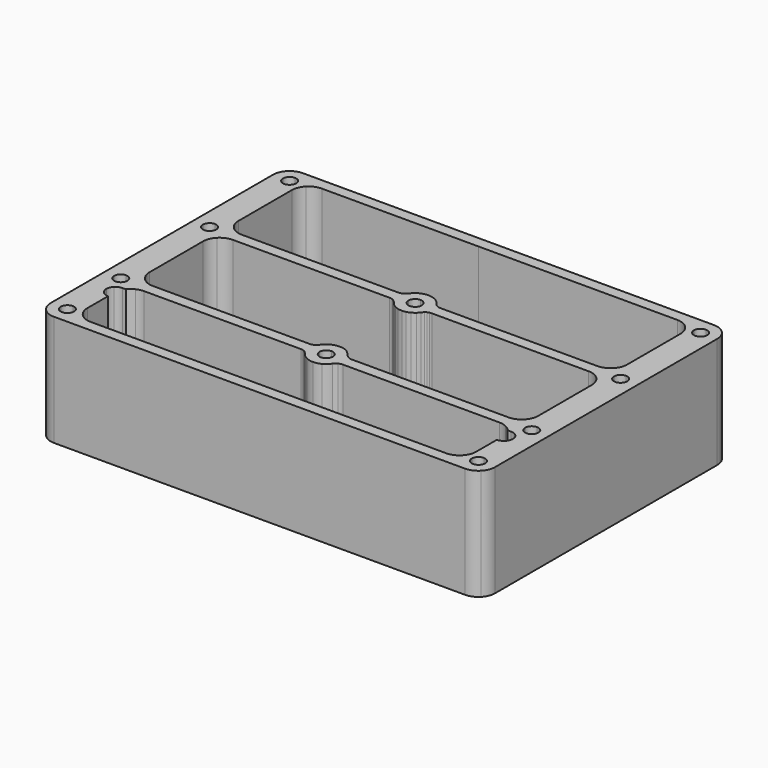
from build123d import *

# Parameters (mm, degrees)
F1_DEPTH = 20


# Not quite as in the source:
# - ends of sketch curves that miss each other by under 0.0002 mm in the source are joined


with BuildPart() as f1:
    # F0 (on Top) → F1 (new body)
    with BuildSketch(Plane.XY):
        with BuildLine():
            Line((-39.999825, 25.00006), (-39.999825, -24.99994))
            Line((-39.999825, -24.99994), (-40.000174, -25.00006))
            ThreePointArc((-40.000174, -25.00006), (-39.771812164, -26.1481105372), (-39.1214940862, -27.1213810862))
            ThreePointArc((-39.1214940862, -27.1213810862), (-38.1480375077, -27.7716732647), (-36.999825, -27.9999399831))
            Line((-36.999825, -27.9999399831), (36.999826, -28.00006))
            ThreePointArc((36.999826, -28.00006), (38.1478759832, -27.7716986429), (39.121146172, -27.121381172))
            ThreePointArc((39.121146172, -27.121381172), (39.7716506494, -26.1480852785), (40.000174978, -24.99994))
            Line((40.000174978, -24.99994), (39.999826, 24.99994))
            ThreePointArc((39.999826, 24.99994), (39.7714639135, 26.1479899431), (39.1211458791, 27.1212598791))
            ThreePointArc((39.1211458791, 27.1212598791), (38.1480624616, 27.7716033194), (37.000175, 28.0000599827))
            Line((37.000175, 28.0000599827), (-37.000174, 27.99994))
            ThreePointArc((-37.000174, 27.99994), (-38.1482239431, 27.7715779135), (-39.1214938791, 27.1212598791))
            ThreePointArc((-39.1214938791, 27.1212598791), (-39.7716257147, 26.1480153964), (-39.999825, 25.00006))
        make_face()
        with BuildLine():
            Line((-38.200174, -24.99956), (-38.199825, -24.99994))
            ThreePointArc((-38.1998249445, -24.99994), (-37.8486064453, -24.1512940355), (-37.000174, -23.7995600552))
            ThreePointArc((-37.000174, -23.79956), (-36.1516455697, -24.1510315697), (-35.800174, -24.99956))
            ThreePointArc((-35.800174, -24.99956), (-36.1516455697, -25.8480884303), (-37.000174, -26.19956))
            ThreePointArc((-37.000174, -26.19956), (-37.8487024303, -25.8480884303), (-38.200174, -24.99956))
        make_face(mode=Mode.SUBTRACT)
        with BuildLine():
            Line((-38.200174, -12.99956), (-38.199825, -12.99994))
            ThreePointArc((-38.1998249445, -12.99994), (-37.8486064453, -12.1512940355), (-37.000174, -11.7995600552))
            ThreePointArc((-37.000174, -11.79956), (-36.1516455697, -12.1510315697), (-35.800174, -12.99956))
            ThreePointArc((-35.800174, -12.99956), (-36.1516455697, -13.8480884303), (-37.000174, -14.19956))
            ThreePointArc((-37.000174, -14.19956), (-37.8487024303, -13.8480884303), (-38.200174, -12.99956))
        make_face(mode=Mode.SUBTRACT)
        with BuildLine():
            Line((-1.200174, -12.99956), (-1.199825, -12.99994))
            ThreePointArc((-1.1998249445, -12.99994), (-0.8486064453, -12.1512940355), (-0.000174, -11.7995600552))
            ThreePointArc((-0.000174, -11.79956), (0.8483544303, -12.1510315697), (1.199826, -12.99956))
            ThreePointArc((1.199826, -12.99956), (0.8483544303, -13.8480884303), (-0.000174, -14.19956))
            ThreePointArc((-0.000174, -14.19956), (-0.8487024303, -13.8480884303), (-1.200174, -12.99956))
        make_face(mode=Mode.SUBTRACT)
        with BuildLine():
            Line((36.603538, -16.75006), (36.603175, -16.74994))
            ThreePointArc((36.603175, -16.74994), (36.4829333909, -17.3619187603), (36.1383180086, -17.8817420086))
            ThreePointArc((36.1383180086, -17.8817420086), (35.6165430962, -18.2356135959), (34.9998259968, -18.3665107942))
            Line((34.9998259968, -18.3665107942), (35.000175, -22.99994))
            ThreePointArc((35.000175, -22.99994), (34.7716506494, -24.1480852785), (34.121146138, -25.1213811381))
            ThreePointArc((34.121146138, -25.1213811381), (33.1478759832, -25.7716986429), (31.999826, -26.00006))
            Line((31.999826, -26.00006), (-31.999825, -25.99994))
            ThreePointArc((-31.999825, -25.99994), (-33.1480375077, -25.7716732647), (-34.1214941324, -25.1213811324))
            ThreePointArc((-34.1214941324, -25.1213811324), (-34.771812164, -24.1481105372), (-35.000174, -23.00006))
            Line((-35.000174, -23.00006), (-34.999825, -18.34994))
            ThreePointArc((-34.999825, -18.34994), (-35.6042335809, -18.2304702332), (-36.1159159305, -17.887302931))
            ThreePointArc((-36.1159159305, -17.887302931), (-36.4642279095, -17.3651332541), (-36.5893969659, -16.7500599998))
            ThreePointArc((-36.5893969659, -16.7500599998), (-36.4636878106, -16.133963155), (-36.1146695958, -15.6109294015))
            ThreePointArc((-36.1146695958, -15.6109294015), (-35.6037340191, -15.2685004223), (-35.0001739964, -15.1500592171))
            Line((-35.0001739964, -15.1500592171), (-34.373825, -15.14994))
            ThreePointArc((-34.373825, -15.14994), (-33.8806261156, -14.6647208591), (-33.2945678918, -14.297000223))
            ThreePointArc((-33.2945678918, -14.297000223), (-32.6642661787, -14.074224434), (-32.0001739998, -13.9974720891))
            Line((-32.0001739998, -13.9974720891), (-3.792825, -13.99294))
            ThreePointArc((-3.792825, -13.99294), (-3.587024283, -14.0085288519), (-3.3845238859, -14.0484105604))
            ThreePointArc((-3.3845238859, -14.0484105604), (-3.1995526999, -14.1089426612), (-3.0236719787, -14.1922759616))
            ThreePointArc((-3.0236719787, -14.1922759616), (-2.8987221408, -14.2721320584), (-2.7848178748, -14.3670808678))
            ThreePointArc((-2.7848178748, -14.3670808678), (-2.6072336828, -14.548031177), (-2.4434346201, -14.7415487017))
            ThreePointArc((-2.4434346201, -14.7415487017), (-1.9532323269, -15.2735515805), (-1.3530931568, -15.6774803045))
            ThreePointArc((-1.3530931568, -15.6774803045), (-0.6961967844, -15.9206969026), (-0.0001739951, -15.999560602))
            ThreePointArc((-0.0001739951, -15.999560602), (0.7201727666, -15.9154593612), (1.3979399526, -15.6573819105))
            ThreePointArc((1.3979399526, -15.6573819105), (1.982334578, -15.2460332249), (2.4460271812, -14.7022374632))
            ThreePointArc((2.4460271812, -14.7022374632), (2.7407409968, -14.4052400968), (3.089711319, -14.1744086099))
            ThreePointArc((3.089711319, -14.1744086099), (3.4350131482, -14.0422107565), (3.8014919924, -13.9931905443))
            Line((3.8014919924, -13.9931905443), (32.000175, -13.99994))
            ThreePointArc((32.000175, -13.99994), (32.6691048373, -14.0761652682), (33.3038019175, -14.3007471693))
            ThreePointArc((33.3038019175, -14.3007471693), (33.8771769518, -14.664706996), (34.3550597723, -15.1472561797))
            Line((34.3550597723, -15.1472561797), (35.003175, -15.14994))
            ThreePointArc((35.003175, -15.14994), (35.6171587026, -15.2707727015), (36.1376999935, -15.6180670065))
            ThreePointArc((36.1376999935, -15.6180670065), (36.4838802077, -16.1374542064), (36.603538, -16.75006))
        make_face(mode=Mode.SUBTRACT)
        with BuildLine():
            Line((35.799826, -24.99956), (35.800175, -24.99994))
            ThreePointArc((35.8001750555, -24.99994), (36.1513935547, -24.1512940355), (36.999826, -23.7995600552))
            ThreePointArc((36.999826, -23.79956), (37.8483544303, -24.1510315697), (38.199826, -24.99956))
            ThreePointArc((38.199826, -24.99956), (37.8483544303, -25.8480884303), (36.999826, -26.19956))
            ThreePointArc((36.999826, -26.19956), (36.1512975697, -25.8480884303), (35.799826, -24.99956))
        make_face(mode=Mode.SUBTRACT)
        with BuildLine():
            Line((34.999826, 2.99994), (35.000175, 3.00006))
            Line((35.000175, 3.00006), (35.000175, -8.99994))
            ThreePointArc((35.000175, -8.99994), (34.7716506494, -10.1480852785), (34.121146138, -11.1213811381))
            ThreePointArc((34.121146138, -11.1213811381), (33.1478759832, -11.7716986429), (31.999826, -12.00006))
            Line((31.999826, -12.00006), (3.810175, -11.99994))
            ThreePointArc((3.810175, -11.99994), (3.4730610862, -11.9616796532), (3.1530679652, -11.8489230717))
            ThreePointArc((3.1530679652, -11.8489230717), (2.833800561, -11.6515843202), (2.5610064723, -11.3937905925))
            ThreePointArc((2.5610064723, -11.3937905925), (2.3088636351, -11.0955933493), (2.037311876, -10.8149561283))
            ThreePointArc((2.037311876, -10.8149561283), (1.8071893103, -10.6107695316), (1.5605320798, -10.4268978829))
            ThreePointArc((1.5605320798, -10.4268978829), (1.4100194875, -10.3334911747), (1.2521070594, -10.2532258697))
            ThreePointArc((1.2521070594, -10.2532258697), (1.064969326, -10.1762092608), (0.8726172571, -10.1133381012))
            ThreePointArc((0.8726172571, -10.1133381012), (0.6668393246, -10.0626764147), (0.4578610603, -10.0274735375))
            ThreePointArc((0.4578610603, -10.0274735375), (0.2293235598, -10.0056398158), (-0.000173999, -9.9995601312))
            ThreePointArc((-0.000173999, -9.9995601312), (-0.7183583445, -10.0837537005), (-1.3940161851, -10.3413656513))
            ThreePointArc((-1.3940161851, -10.3413656513), (-2.0176152889, -10.7733522055), (-2.5231648411, -11.3389561115))
            ThreePointArc((-2.5231648411, -11.3389561115), (-2.7518538477, -11.6084835939), (-3.0417751614, -11.81069469))
            ThreePointArc((-3.0417751614, -11.81069469), (-3.4064030036, -11.949362238), (-3.7931999932, -12.0000604896))
            Line((-3.7931999932, -12.0000604896), (-31.999825, -11.99994))
            ThreePointArc((-31.999825, -11.99994), (-33.1480375077, -11.7716732647), (-34.1214941324, -11.1213811324))
            ThreePointArc((-34.1214941324, -11.1213811324), (-34.771812164, -10.1481105372), (-35.000174, -9.00006))
            Line((-35.000174, -9.00006), (-34.999825, 3.00006))
            ThreePointArc((-34.999825, 3.00006), (-34.7716257147, 4.1480153964), (-34.1214942965, 5.1212602964))
            ThreePointArc((-34.1214942965, 5.1212602964), (-33.1482239431, 5.7715779135), (-32.000174, 5.99994))
            Line((-32.000174, 5.99994), (-3.792825, 6.00006))
            ThreePointArc((-3.792825, 6.00006), (-3.4284357853, 5.9550527167), (-3.0858729784, 5.8229320405))
            ThreePointArc((-3.0858729784, 5.8229320405), (-2.7370107339, 5.5859262528), (-2.4460229877, 5.2806350094))
            ThreePointArc((-2.4460229877, 5.2806350094), (-2.2554634836, 5.0183904427), (-2.0288070694, 4.7866319214))
            ThreePointArc((-2.0288070694, 4.7866319214), (-1.7197815139, 4.5450969451), (-1.3839962662, 4.3424044923))
            ThreePointArc((-1.3839962662, 4.3424044923), (-1.0626971467, 4.1978569726), (-0.7263699901, 4.0929230402))
            ThreePointArc((-0.7263699901, 4.0929230402), (-0.3659475679, 4.0256723979), (-0.0001740023, 4.0004397915))
            ThreePointArc((-0.0001740023, 4.0004397915), (0.3494281759, 4.0205254152), (0.6941079837, 4.0823390675))
            ThreePointArc((0.6941079837, 4.0823390675), (1.031369758, 4.1855874283), (1.353961138, 4.3282077323))
            ThreePointArc((1.353961138, 4.3282077323), (1.6950242622, 4.5305551779), (2.00960672, 4.7720223229))
            ThreePointArc((2.00960672, 4.7720223229), (2.2489162642, 5.0107950752), (2.4525529704, 5.2806350193))
            ThreePointArc((2.4525529704, 5.2806350193), (2.6118008292, 5.4657092745), (2.7875919965, 5.635149004))
            ThreePointArc((2.7875919965, 5.635149004), (2.9317797973, 5.7465375496), (3.0887516635, 5.8390436626))
            ThreePointArc((3.0887516635, 5.8390436626), (3.2486759708, 5.9080369394), (3.4159650383, 5.9565158284))
            ThreePointArc((3.4159650383, 5.9565158284), (3.6118561345, 5.9890512814), (3.810132, 5.99994))
            Line((3.810132, 5.99994), (32.000175, 6.00006))
            ThreePointArc((32.000175, 6.00006), (33.1480624616, 5.7716033194), (34.1211461017, 5.1212601017))
            ThreePointArc((34.1211461017, 5.1212601017), (34.7714639135, 4.1479899431), (34.999826, 2.99994))
        make_face(mode=Mode.SUBTRACT)
        with BuildLine():
            Line((35.799826, -12.99956), (35.800175, -12.99994))
            ThreePointArc((35.8001750555, -12.99994), (36.1513935547, -12.1512940355), (36.999826, -11.7995600552))
            ThreePointArc((36.999826, -11.79956), (37.8483544303, -12.1510315697), (38.199826, -12.99956))
            ThreePointArc((38.199826, -12.99956), (37.8483544303, -13.8480884303), (36.999826, -14.19956))
            ThreePointArc((36.999826, -14.19956), (36.1512975697, -13.8480884303), (35.799826, -12.99956))
        make_face(mode=Mode.SUBTRACT)
        with BuildLine():
            Line((-38.200174, 7.00044), (-38.199825, 7.00006))
            ThreePointArc((-38.1998249445, 7.00006), (-37.8486064453, 7.8487059645), (-37.000174, 8.2004399448))
            ThreePointArc((-37.000174, 8.20044), (-36.1516455697, 7.8489684303), (-35.800174, 7.00044))
            ThreePointArc((-35.800174, 7.00044), (-36.1516455697, 6.1519115697), (-37.000174, 5.80044))
            ThreePointArc((-37.000174, 5.80044), (-37.8487024303, 6.1519115697), (-38.200174, 7.00044))
        make_face(mode=Mode.SUBTRACT)
        with BuildLine():
            Line((-1.200174, 7.00044), (-1.199825, 7.00006))
            ThreePointArc((-1.1998249445, 7.00006), (-0.8486064453, 7.8487059645), (-0.000174, 8.2004399448))
            ThreePointArc((-0.000174, 8.20044), (0.8483544303, 7.8489684303), (1.199826, 7.00044))
            ThreePointArc((1.199826, 7.00044), (0.8483544303, 6.1519115697), (-0.000174, 5.80044))
            ThreePointArc((-0.000174, 5.80044), (-0.8487024303, 6.1519115697), (-1.200174, 7.00044))
        make_face(mode=Mode.SUBTRACT)
        with BuildLine():
            Line((-38.200174, 24.99994), (-38.199825, 25.00006))
            ThreePointArc((-38.1998249945, 25.00006), (-37.8485029272, 25.8484559997), (-37.000174, 26.1999399946))
            ThreePointArc((-37.000174, 26.19994), (-36.1516455697, 25.8484684303), (-35.800174, 24.99994))
            ThreePointArc((-35.800174, 24.99994), (-36.1516455697, 24.1514115697), (-37.000174, 23.79994))
            ThreePointArc((-37.000174, 23.79994), (-37.8487024303, 24.1514115697), (-38.200174, 24.99994))
        make_face(mode=Mode.SUBTRACT)
        with BuildLine():
            Line((35.799826, 7.00044), (35.800175, 7.00006))
            ThreePointArc((35.8001750555, 7.00006), (36.1513935547, 7.8487059645), (36.999826, 8.2004399448))
            ThreePointArc((36.999826, 8.20044), (37.8483544303, 7.8489684303), (38.199826, 7.00044))
            ThreePointArc((38.199826, 7.00044), (37.8483544303, 6.1519115697), (36.999826, 5.80044))
            ThreePointArc((36.999826, 5.80044), (36.1512975697, 6.1519115697), (35.799826, 7.00044))
        make_face(mode=Mode.SUBTRACT)
        with BuildLine():
            Line((34.999826, 22.99994), (35.000175, 23.00006))
            Line((35.000175, 23.00006), (35.000175, 11.00006))
            ThreePointArc((35.000175, 11.00006), (34.7716506494, 9.8519147215), (34.121146138, 8.8786188619))
            ThreePointArc((34.121146138, 8.8786188619), (33.1478759832, 8.2283013571), (31.999826, 7.99994))
            Line((31.999826, 7.99994), (3.810175, 8.00006))
            ThreePointArc((3.810175, 8.00006), (3.4235803672, 8.0454859973), (3.0588864169, 8.1815638062))
            ThreePointArc((3.0588864169, 8.1815638062), (2.7497243033, 8.394045477), (2.5026107087, 8.6762948031))
            ThreePointArc((2.5026107087, 8.6762948031), (2.0284709982, 9.2275913259), (1.4329928055, 9.6448946323))
            ThreePointArc((1.4329928055, 9.6448946323), (0.7381569449, 9.9103292728), (-0.000174, 10.0004398779))
            ThreePointArc((-0.000174, 10.0004398779), (-0.3694274886, 9.9797063181), (-0.7330550376, 9.9122301492))
            ThreePointArc((-0.7330550376, 9.9122301492), (-1.0971549856, 9.7960856126), (-1.4442170202, 9.6360660376))
            ThreePointArc((-1.4442170202, 9.6360660376), (-1.76672104, 9.4359987043), (-2.0621862991, 9.1978053275))
            ThreePointArc((-2.0621862991, 9.1978053275), (-2.3015387887, 8.9475337569), (-2.5049799594, 8.6672889746))
            ThreePointArc((-2.5049799594, 8.6672889746), (-2.6502064138, 8.4994918359), (-2.812037178, 8.3476452106))
            ThreePointArc((-2.812037178, 8.3476452106), (-2.9626572369, 8.2354346871), (-3.1258878041, 8.1425186007))
            ThreePointArc((-3.1258878041, 8.1425186007), (-3.2424323815, 8.0939718893), (-3.364045832, 8.0600662139))
            ThreePointArc((-3.364045832, 8.0600662139), (-3.5775508268, 8.0223509144), (-3.7932000078, 7.9999401152))
            Line((-3.7932000078, 7.9999401152), (-31.999825, 8.00006))
            ThreePointArc((-31.999825, 8.00006), (-33.1480375077, 8.2283267353), (-34.1214941324, 8.8786188676))
            ThreePointArc((-34.1214941324, 8.8786188676), (-34.771812164, 9.8518894628), (-35.000174, 10.99994))
            Line((-35.000174, 10.99994), (-34.999825, 23.00006))
            ThreePointArc((-34.999825, 23.00006), (-34.7716257147, 24.1480153964), (-34.1214942965, 25.1212602964))
            ThreePointArc((-34.1214942965, 25.1212602964), (-33.1482239431, 25.7715779135), (-32.000174, 25.99994))
            Line((-32.000174, 25.99994), (-3.796825, 26.00006))
            Line((-3.796825, 26.00006), (-2.349825, 26.00006))
            Line((-2.349825, 26.00006), (-0.168825, 26.00006))
            Line((-0.168825, 26.00006), (2.628175, 26.00006))
            Line((2.628175, 26.00006), (3.933175, 26.00006))
            Line((3.933175, 26.00006), (32.000175, 26.00006))
            ThreePointArc((32.000175, 26.00006), (33.1480624616, 25.7716033194), (34.1211461017, 25.1212601017))
            ThreePointArc((34.1211461017, 25.1212601017), (34.7714639135, 24.1479899431), (34.999826, 22.99994))
        make_face(mode=Mode.SUBTRACT)
        with BuildLine():
            Line((35.799826, 24.99994), (35.800175, 25.00006))
            ThreePointArc((35.8001750055, 25.00006), (36.1514970728, 25.8484559997), (36.999826, 26.1999399946))
            ThreePointArc((36.999826, 26.19994), (37.8483544303, 25.8484684303), (38.199826, 24.99994))
            ThreePointArc((38.199826, 24.99994), (37.8483544303, 24.1514115697), (36.999826, 23.79994))
            ThreePointArc((36.999826, 23.79994), (36.1512975697, 24.1514115697), (35.799826, 24.99994))
        make_face(mode=Mode.SUBTRACT)
    extrude(amount=F1_DEPTH)


solid = f1.part
